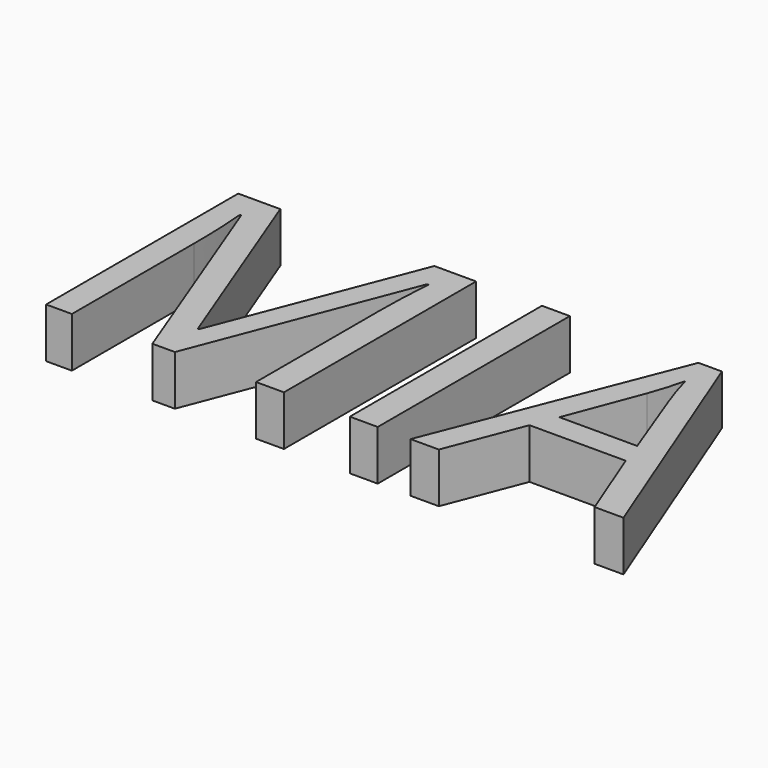
from build123d import *

# Parameters (mm, degrees)
F0_TEXT_SIZE = 85.5820512192
F1_DEPTH     = 12.7


# Not quite as in the source:
# - Text() gives the source's letters only with a copy of the font that has no kerning and outlines rounded to 1/6400 em; it was checked with that copy


with BuildPart() as f1:
    # F0 (on Top) → F1 (new body)
    with BuildSketch(Plane.XY):
        with Locations((-76.5024516732, -27.7759842575)):
            Text('MIA', F0_TEXT_SIZE, font='Open Sans', text_align=(TextAlign.LEFT, TextAlign.BOTTOM))
    extrude(amount=F1_DEPTH)


solid = f1.part
